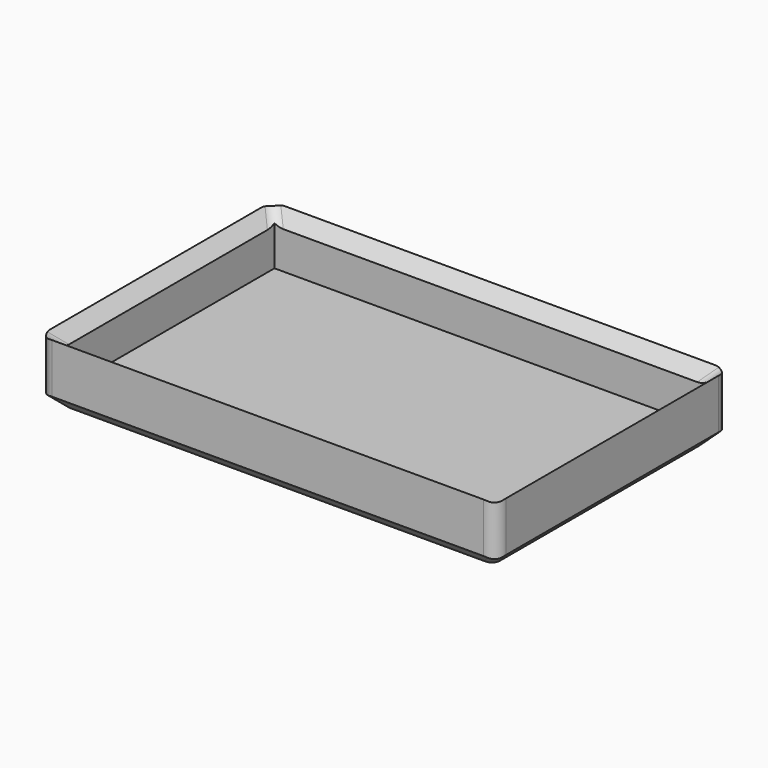
from build123d import *

# Parameters (mm, degrees)
F0_W         = 110
F0_H         = 70
F1_DEPTH     = 15
F2_T         = -3
F3_SIZE      = 3
F4_SIZE      = 2.99999
F5_T4_DEPTH  = 13.85638914
F5_T11_DEPTH = 13.85638914
F5_T17_DEPTH = 13.85638914
F5_T23_DEPTH = 13.85638914
F5_T30_DEPTH = 13.85638914
F5_T36_DEPTH = 13.85638914
F5_T42_DEPTH = 13.85638914
F5_T49_DEPTH = 13.85638914
F5_T55_DEPTH = 13.85638914
F5_T61_DEPTH = 13.85638914
F5_T68_DEPTH = 13.85638914
F5_T74_DEPTH = 13.85638914
F5_T77_DEPTH = 27
F5_T79_DEPTH = 13.8564064606
F5_T81_DEPTH = 13.8564064606
F5_T83_DEPTH = 13.8564064606
F5_T85_DEPTH = 13.8564064606


# Not quite as in the source:
# - a fillet or chamfer that OpenCascade refuses, or shapes differently, is made with other operations: its cross-section is extruded or revolved along the edge and cut away or added
# - a fillet or chamfer is up to 0.001 mm smaller than in the source, because OpenCascade refuses the exact size


with BuildPart() as f1:
    # F0 (on Top) → F1 (new body)
    with BuildSketch(Plane.XY):
        with Locations((12.2063489258, -6.1995962761)):
            Rectangle(F0_W, F0_H)
    extrude(amount=F1_DEPTH)

    # F2
    f2_openings = [f1.faces().sort_by_distance(p)[0] for p in [
        (12.206349, -6.199596, 15),
    ]]
    offset(amount=F2_T, openings=f2_openings)

    # F3
    f3_edges = [f1.edges().sort_by_distance(p)[0] for p in [
        (-42.793651, -6.199596, 0),
        (12.206349, -41.199596, 0),
        (67.206349, -6.199596, 0),
        (12.206349, 28.800404, 0),
    ]]
    chamfer(f3_edges, length=F3_SIZE)

    # F4 (size 3 in the source; OpenCascade refuses exactly that, so slightly less here)
    f4_edges = [f1.edges().sort_by_distance(p)[0] for p in [
        (12.206349, 25.800404, 15),
        (-39.793651, -6.199596, 15),
        (64.206349, -6.199596, 15),
        (12.206349, -38.199596, 15),
    ]]
    chamfer(f4_edges, length=F4_SIZE)

    # F5: fillet of radius 3 on 12 edges, made by hand


with BuildPart() as f5_tool2:
    # F5_s3 → F5_t4 (new body)
    with BuildSketch(Plane(origin=(43.6353084006, -43.6353084006, 43.6353084006), x_dir=(-0.7071067812, -0.7071067812, 0), z_dir=(-0.5773502692, 0.5773502692, -0.5773502692))):
        with BuildLine():
            ThreePointArc((-19.8895511553, -31.1430595221), (-18.3895511553, -31.5449833108), (-16.8895511553, -31.1430595221))
            Line((-16.8895511553, -31.1430595221), (-18.3895511553, -32.0090849259))
            Line((-18.3895511553, -32.0090849259), (-19.8895511553, -31.1430595221))
        make_face()
    extrude(amount=F5_T4_DEPTH)

    split(bisect_by=Plane.XY.offset(15), keep=Keep.BOTTOM)

    split(bisect_by=Plane.YZ.offset(64.2063489258), keep=Keep.TOP)

    split(bisect_by=Plane.XZ.offset(38.1995962761), keep=Keep.TOP)


with BuildPart() as f1_1:
    add(f1.part)

    # F5_t1: union F5_tool2
    add(f5_tool2.part)


with BuildPart() as f5_tool9:
    # F5_s10 → F5_t11 (new body)
    with BuildSketch(Plane(origin=(43.6353084006, -43.6353084006, 43.6353084006), x_dir=(-0.7071067812, -0.7071067812, 0), z_dir=(-0.5773502692, 0.5773502692, -0.5773502692))):
        with BuildLine():
            ThreePointArc((-19.8895511553, -31.1430595221), (-18.3895511553, -31.5449833108), (-16.8895511553, -31.1430595221))
            Line((-16.8895511553, -31.1430595221), (-18.3895511553, -32.0090849259))
            Line((-18.3895511553, -32.0090849259), (-19.8895511553, -31.1430595221))
        make_face()
    extrude(amount=F5_T11_DEPTH)

    split(bisect_by=Plane.YZ.offset(64.2063489258), keep=Keep.BOTTOM)

    split(bisect_by=Plane.XZ.offset(38.1995962761), keep=Keep.TOP)


with BuildPart() as f1_2:
    add(f1_1.part)

    # F5_t8: union F5_tool9
    add(f5_tool9.part)


with BuildPart() as f5_tool15:
    # F5_s16 → F5_t17 (new body)
    with BuildSketch(Plane(origin=(43.6353084006, -43.6353084006, 43.6353084006), x_dir=(-0.7071067812, -0.7071067812, 0), z_dir=(-0.5773502692, 0.5773502692, -0.5773502692))):
        with BuildLine():
            ThreePointArc((-19.8895511553, -31.1430595221), (-18.3895511553, -31.5449833108), (-16.8895511553, -31.1430595221))
            Line((-16.8895511553, -31.1430595221), (-18.3895511553, -32.0090849259))
            Line((-18.3895511553, -32.0090849259), (-19.8895511553, -31.1430595221))
        make_face()
    extrude(amount=F5_T17_DEPTH)

    split(bisect_by=Plane.YZ.offset(64.2063489258), keep=Keep.TOP)

    split(bisect_by=Plane.XZ.offset(38.1995962761), keep=Keep.BOTTOM)


with BuildPart() as f1_3:
    add(f1_2.part)

    # F5_t14: union F5_tool15
    add(f5_tool15.part)


with BuildPart() as f5_tool21:
    # F5_s22 → F5_t23 (new body)
    with BuildSketch(Plane(origin=(-35.4977424501, -35.4977424501, 35.4977424501), x_dir=(-0.7071067812, 0.7071067812, 0), z_dir=(0.5773502692, 0.5773502692, -0.5773502692))):
        with BuildLine():
            ThreePointArc((2.6271669573, -21.1766173586), (1.1271669573, -21.5785411472), (-0.3728330427, -21.1766173586))
            Line((-0.3728330427, -21.1766173586), (1.1271669573, -22.0426427624))
            Line((1.1271669573, -22.0426427624), (2.6271669573, -21.1766173586))
        make_face()
    extrude(amount=F5_T23_DEPTH)

    split(bisect_by=Plane.XY.offset(15), keep=Keep.BOTTOM)

    split(bisect_by=Plane.YZ.offset(-39.7936510742), keep=Keep.BOTTOM)

    split(bisect_by=Plane.XZ.offset(38.1995962761), keep=Keep.TOP)


with BuildPart() as f1_4:
    add(f1_3.part)

    # F5_t20: union F5_tool21
    add(f5_tool21.part)


with BuildPart() as f5_tool28:
    # F5_s29 → F5_t30 (new body)
    with BuildSketch(Plane(origin=(-35.4977424501, -35.4977424501, 35.4977424501), x_dir=(-0.7071067812, 0.7071067812, 0), z_dir=(0.5773502692, 0.5773502692, -0.5773502692))):
        with BuildLine():
            ThreePointArc((2.6271669573, -21.1766173586), (1.1271669573, -21.5785411472), (-0.3728330427, -21.1766173586))
            Line((-0.3728330427, -21.1766173586), (1.1271669573, -22.0426427624))
            Line((1.1271669573, -22.0426427624), (2.6271669573, -21.1766173586))
        make_face()
    extrude(amount=F5_T30_DEPTH)

    split(bisect_by=Plane.YZ.offset(-39.7936510742), keep=Keep.TOP)

    split(bisect_by=Plane.XZ.offset(38.1995962761), keep=Keep.TOP)


with BuildPart() as f1_5:
    add(f1_4.part)

    # F5_t27: union F5_tool28
    add(f5_tool28.part)


with BuildPart() as f5_tool34:
    # F5_s35 → F5_t36 (new body)
    with BuildSketch(Plane(origin=(-35.4977424501, -35.4977424501, 35.4977424501), x_dir=(-0.7071067812, 0.7071067812, 0), z_dir=(0.5773502692, 0.5773502692, -0.5773502692))):
        with BuildLine():
            ThreePointArc((2.6271669573, -21.1766173586), (1.1271669573, -21.5785411472), (-0.3728330427, -21.1766173586))
            Line((-0.3728330427, -21.1766173586), (1.1271669573, -22.0426427624))
            Line((1.1271669573, -22.0426427624), (2.6271669573, -21.1766173586))
        make_face()
    extrude(amount=F5_T36_DEPTH)

    split(bisect_by=Plane.YZ.offset(-39.7936510742), keep=Keep.BOTTOM)

    split(bisect_by=Plane.XZ.offset(38.1995962761), keep=Keep.BOTTOM)


with BuildPart() as f1_6:
    add(f1_5.part)

    # F5_t33: union F5_tool34
    add(f5_tool34.part)


with BuildPart() as f5_tool40:
    # F5_s41 → F5_t42 (new body)
    with BuildSketch(Plane(origin=(-31.364678266, 31.364678266, 31.364678266), x_dir=(0.7071067812, 0.7071067812, 0), z_dir=(0.5773502692, -0.5773502692, -0.5773502692))):
        with BuildLine():
            ThreePointArc((-8.3947200922, -16.114668196), (-9.8947200922, -16.5165919847), (-11.3947200922, -16.114668196))
            Line((-11.3947200922, -16.114668196), (-9.8947200922, -16.9806935998))
            Line((-9.8947200922, -16.9806935998), (-8.3947200922, -16.114668196))
        make_face()
    extrude(amount=F5_T42_DEPTH)

    split(bisect_by=Plane.XY.offset(15), keep=Keep.BOTTOM)

    split(bisect_by=Plane.XZ.offset(-25.8004037239), keep=Keep.BOTTOM)

    split(bisect_by=Plane.YZ.offset(-39.7936510742), keep=Keep.BOTTOM)


with BuildPart() as f1_7:
    add(f1_6.part)

    # F5_t39: union F5_tool40
    add(f5_tool40.part)


with BuildPart() as f5_tool47:
    # F5_s48 → F5_t49 (new body)
    with BuildSketch(Plane(origin=(-31.364678266, 31.364678266, 31.364678266), x_dir=(0.7071067812, 0.7071067812, 0), z_dir=(0.5773502692, -0.5773502692, -0.5773502692))):
        with BuildLine():
            ThreePointArc((-8.3947200922, -16.114668196), (-9.8947200922, -16.5165919847), (-11.3947200922, -16.114668196))
            Line((-11.3947200922, -16.114668196), (-9.8947200922, -16.9806935998))
            Line((-9.8947200922, -16.9806935998), (-8.3947200922, -16.114668196))
        make_face()
    extrude(amount=F5_T49_DEPTH)

    split(bisect_by=Plane.XZ.offset(-25.8004037239), keep=Keep.TOP)

    split(bisect_by=Plane.YZ.offset(-39.7936510742), keep=Keep.BOTTOM)


with BuildPart() as f1_8:
    add(f1_7.part)

    # F5_t46: union F5_tool47
    add(f5_tool47.part)


with BuildPart() as f5_tool53:
    # F5_s54 → F5_t55 (new body)
    with BuildSketch(Plane(origin=(-31.364678266, 31.364678266, 31.364678266), x_dir=(0.7071067812, 0.7071067812, 0), z_dir=(0.5773502692, -0.5773502692, -0.5773502692))):
        with BuildLine():
            ThreePointArc((-8.3947200922, -16.114668196), (-9.8947200922, -16.5165919847), (-11.3947200922, -16.114668196))
            Line((-11.3947200922, -16.114668196), (-9.8947200922, -16.9806935998))
            Line((-9.8947200922, -16.9806935998), (-8.3947200922, -16.114668196))
        make_face()
    extrude(amount=F5_T55_DEPTH)

    split(bisect_by=Plane.XZ.offset(-25.8004037239), keep=Keep.BOTTOM)

    split(bisect_by=Plane.YZ.offset(-39.7936510742), keep=Keep.TOP)


with BuildPart() as f1_9:
    add(f1_8.part)

    # F5_t52: union F5_tool53
    add(f5_tool53.part)


with BuildPart() as f5_tool59:
    # F5_s60 → F5_t61 (new body)
    with BuildSketch(Plane(origin=(39.5022442166, 39.5022442166, 39.5022442166), x_dir=(0.7071067812, -0.7071067812, 0), z_dir=(-0.5773502692, -0.5773502692, -0.5773502692))):
        with BuildLine():
            ThreePointArc((25.6571042902, -26.0811103596), (27.1571042902, -26.4830341482), (28.6571042902, -26.0811103596))
            Line((28.6571042902, -26.0811103596), (27.1571042902, -26.9471357634))
            Line((27.1571042902, -26.9471357634), (25.6571042902, -26.0811103596))
        make_face()
    extrude(amount=F5_T61_DEPTH)

    split(bisect_by=Plane.XY.offset(15), keep=Keep.BOTTOM)

    split(bisect_by=Plane.XZ.offset(-25.8004037239), keep=Keep.BOTTOM)

    split(bisect_by=Plane.YZ.offset(64.2063489258), keep=Keep.TOP)


with BuildPart() as f1_10:
    add(f1_9.part)

    # F5_t58: union F5_tool59
    add(f5_tool59.part)


with BuildPart() as f5_tool66:
    # F5_s67 → F5_t68 (new body)
    with BuildSketch(Plane(origin=(39.5022442166, 39.5022442166, 39.5022442166), x_dir=(0.7071067812, -0.7071067812, 0), z_dir=(-0.5773502692, -0.5773502692, -0.5773502692))):
        with BuildLine():
            ThreePointArc((25.6571042902, -26.0811103596), (27.1571042902, -26.4830341482), (28.6571042902, -26.0811103596))
            Line((28.6571042902, -26.0811103596), (27.1571042902, -26.9471357634))
            Line((27.1571042902, -26.9471357634), (25.6571042902, -26.0811103596))
        make_face()
    extrude(amount=F5_T68_DEPTH)

    split(bisect_by=Plane.XZ.offset(-25.8004037239), keep=Keep.TOP)

    split(bisect_by=Plane.YZ.offset(64.2063489258), keep=Keep.TOP)


with BuildPart() as f1_11:
    add(f1_10.part)

    # F5_t65: union F5_tool66
    add(f5_tool66.part)


with BuildPart() as f5_tool72:
    # F5_s73 → F5_t74 (new body)
    with BuildSketch(Plane(origin=(39.5022442166, 39.5022442166, 39.5022442166), x_dir=(0.7071067812, -0.7071067812, 0), z_dir=(-0.5773502692, -0.5773502692, -0.5773502692))):
        with BuildLine():
            ThreePointArc((25.6571042902, -26.0811103596), (27.1571042902, -26.4830341482), (28.6571042902, -26.0811103596))
            Line((28.6571042902, -26.0811103596), (27.1571042902, -26.9471357634))
            Line((27.1571042902, -26.9471357634), (25.6571042902, -26.0811103596))
        make_face()
    extrude(amount=F5_T74_DEPTH)

    split(bisect_by=Plane.XZ.offset(-25.8004037239), keep=Keep.BOTTOM)

    split(bisect_by=Plane.YZ.offset(64.2063489258), keep=Keep.BOTTOM)


with BuildPart() as f1_12:
    add(f1_11.part)

    # F5_t71: union F5_tool72
    add(f5_tool72.part)

    # F5_s78 → F5_t77 (cut)
    with BuildSketch(Plane.XY.offset(-4.5)):
        with BuildLine():
            ThreePointArc((67.2063489258, -38.1995962761), (66.3276692694, -40.3209166197), (64.2063489258, -41.1995962761))
            Line((64.2063489258, -41.1995962761), (67.2063489258, -41.1995962761))
            Line((67.2063489258, -41.1995962761), (67.2063489258, -38.1995962761))
        make_face()
        with BuildLine():
            ThreePointArc((-39.7936510742, -41.1995962761), (-41.9149714177, -40.3209166197), (-42.7936510742, -38.1995962761))
            Line((-42.7936510742, -38.1995962761), (-42.7936510742, -41.1995962761))
            Line((-42.7936510742, -41.1995962761), (-39.7936510742, -41.1995962761))
        make_face()
        with BuildLine():
            ThreePointArc((64.2063489258, 28.8004037239), (66.3276692694, 27.9217240674), (67.2063489258, 25.8004037239))
            Line((67.2063489258, 25.8004037239), (67.2063489258, 28.8004037239))
            Line((67.2063489258, 28.8004037239), (64.2063489258, 28.8004037239))
        make_face()
        with BuildLine():
            ThreePointArc((-39.7936510742, 28.8004037239), (-41.9149714177, 27.9217240674), (-42.7936510742, 25.8004037239))
            Line((-42.7936510742, 25.8004037239), (-42.7936510742, 28.8004037239))
            Line((-42.7936510742, 28.8004037239), (-39.7936510742, 28.8004037239))
        make_face()
    extrude(amount=F5_T77_DEPTH, mode=Mode.SUBTRACT)

    # F5_s80 → F5_t79 (cut)
    with BuildSketch(Plane(origin=(-31.4977491168, -31.4977491168, 31.4977491168), x_dir=(-0.7071067812, 0.7071067812, 0), z_dir=(0.5773502692, 0.5773502692, -0.5773502692))):
        with BuildLine():
            ThreePointArc((2.6271669573, -30.9745844947), (1.1271669573, -31.3765082833), (-0.3728330427, -30.9745844947))
            Line((-0.3728330427, -30.9745844947), (1.1271669573, -31.8406098985))
            Line((1.1271669573, -31.8406098985), (2.6271669573, -30.9745844947))
        make_face()
    extrude(amount=F5_T79_DEPTH, mode=Mode.SUBTRACT)

    # F5_s82 → F5_t81 (cut)
    with BuildSketch(Plane(origin=(-27.3646849327, 27.3646849327, 27.3646849327), x_dir=(0.7071067812, 0.7071067812, 0), z_dir=(0.5773502692, -0.5773502692, -0.5773502692))):
        with BuildLine():
            ThreePointArc((-8.3947200922, -25.9126353321), (-9.8947200922, -26.3145591208), (-11.3947200922, -25.9126353321))
            Line((-11.3947200922, -25.9126353321), (-9.8947200922, -26.7786607359))
            Line((-9.8947200922, -26.7786607359), (-8.3947200922, -25.9126353321))
        make_face()
    extrude(amount=F5_T81_DEPTH, mode=Mode.SUBTRACT)

    # F5_s84 → F5_t83 (cut)
    with BuildSketch(Plane(origin=(39.6353150673, -39.6353150673, 39.6353150673), x_dir=(-0.7071067812, -0.7071067812, 0), z_dir=(-0.5773502692, 0.5773502692, -0.5773502692))):
        with BuildLine():
            ThreePointArc((-16.8895511553, -40.9410266582), (-18.3895511553, -41.3429504469), (-19.8895511553, -40.9410266582))
            Line((-19.8895511553, -40.9410266582), (-18.3895511553, -41.807052062))
            Line((-18.3895511553, -41.807052062), (-16.8895511553, -40.9410266582))
        make_face()
    extrude(amount=F5_T83_DEPTH, mode=Mode.SUBTRACT)

    # F5_s86 → F5_t85 (cut)
    with BuildSketch(Plane(origin=(35.5022508832, 35.5022508832, 35.5022508832), x_dir=(0.7071067812, -0.7071067812, 0), z_dir=(-0.5773502692, -0.5773502692, -0.5773502692))):
        with BuildLine():
            ThreePointArc((25.6571042902, -35.8790774957), (27.1571042902, -36.2810012843), (28.6571042902, -35.8790774957))
            Line((28.6571042902, -35.8790774957), (27.1571042902, -36.7451028995))
            Line((27.1571042902, -36.7451028995), (25.6571042902, -35.8790774957))
        make_face()
    extrude(amount=F5_T85_DEPTH, mode=Mode.SUBTRACT)


solid = f1_12.part
